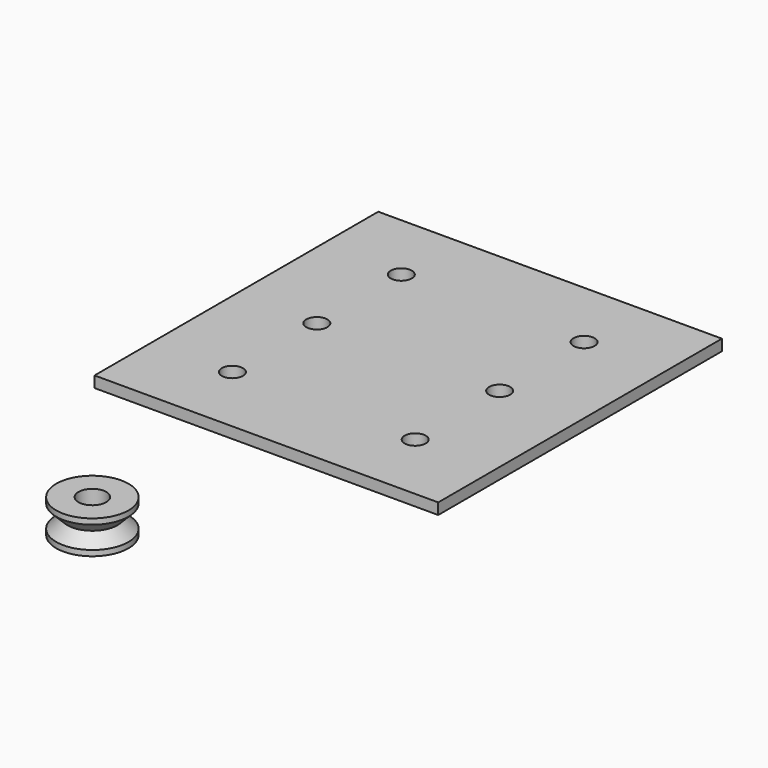
from build123d import *

# Parameters (mm, degrees)
F0_W     = 61.8
F0_H     = 100.8965958967
F1_DEPTH = 5
F4_R     = 1.9
F4_W     = 61.8
F4_H     = 18.5648719378
F5_DEPTH = 25
F7_DEPTH = 3


with BuildPart() as f1:
    # F0 (on Top) → F1 (new body)
    with BuildSketch(Plane.XY):
        Rectangle(F0_W, F0_H)
    extrude(amount=F1_DEPTH)

    # F4 (on face) → F5 (cut)
    with BuildSketch(Plane.XY.offset(5)):
        with Locations((-16.4355339059, 0)):
            Circle(F4_R)
        with Locations((-16.4355339059, -18.9781198497)):
            Circle(F4_R)
        with Locations((16.4355339059, 18.9781198497)):
            Circle(F4_R)
        with Locations((16.4355339059, 0)):
            Circle(F4_R)
        with Locations((16.4355339059, -18.9781198497)):
            Circle(F4_R)
        with Locations((-16.4355339059, 18.9781198497)):
            Circle(F4_R)
        with Locations((0, 41.1658619795)):
            Rectangle(F4_W, F4_H)
        with Locations((0, -41.1658619795)):
            Rectangle(F4_W, F4_H)
    extrude(amount=-F5_DEPTH, mode=Mode.SUBTRACT)

    # F7 (cut): a face of the model
    f7_faces = [f1.faces().sort_by_distance(p)[0] for p in [
        (0, 0, 0),
    ]]
    extrude(f7_faces, amount=-F7_DEPTH, mode=Mode.SUBTRACT)


with BuildPart() as f3:
    # F2 (on face) → F3 (revolve)
    with BuildSketch(Plane.XZ.offset(50.4482979484)):
        Polygon((-9.9355339059, -2), (-13.9355339059, -2), (-13.9355339059, -8), (-9.9355339059, -8), (-9.9355339059, -7), (-11.9355339059, -5), (-9.9355339059, -3), align=None)
    revolve(axis=Axis((-16.4355339059, -50.4482979484, -5), (0, 0, -1)))


solid = Compound([f1.part, f3.part])
